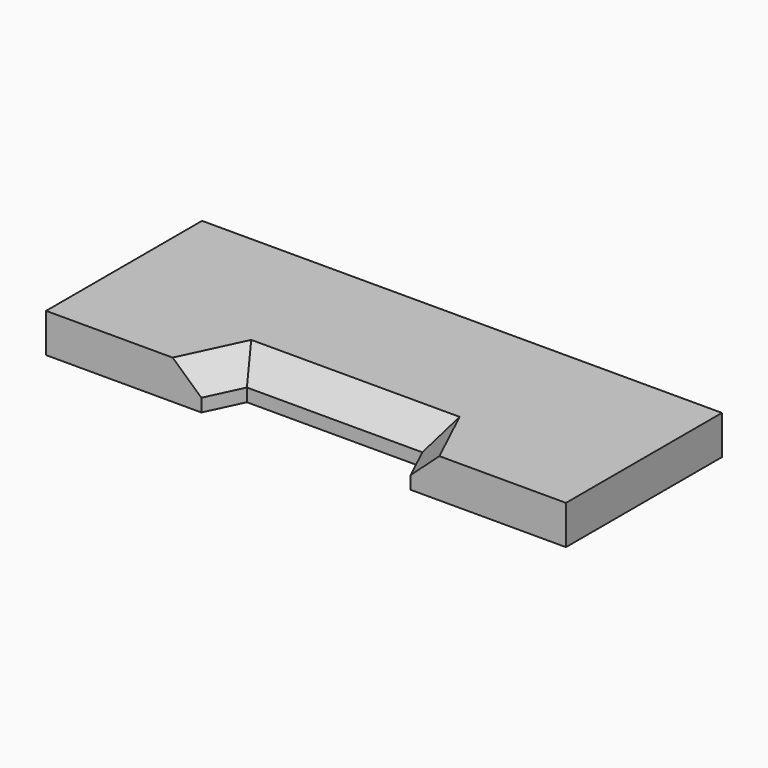
from build123d import *

# Parameters (mm, degrees)
F1_DEPTH = 3
F2_SIZE  = 2


# Not quite as in the source:
# - a feature names something its author has since deleted; it is built from what else it names


with BuildPart() as f1:
    # F0 (on Top) → F1 (new body)
    with BuildSketch(Plane.XY):
        Polygon((8.05, -7.5), (20, -7.5), (20, 7.5), (-20, 7.5), (-20, -7.5), (-8.05, -7.5), (-6.75, -4.75), (0, -4.75), (6.75, -4.75), align=None)
    extrude(amount=F1_DEPTH)

    # F2
    f2_edges = [f1.edges().sort_by_distance(p)[0] for p in [
        (-7.4, -6.125, 3),
        (0, -4.75, 3),
        (7.4, -6.125, 3),
    ]]
    chamfer(f2_edges, length=F2_SIZE)


solid = f1.part
